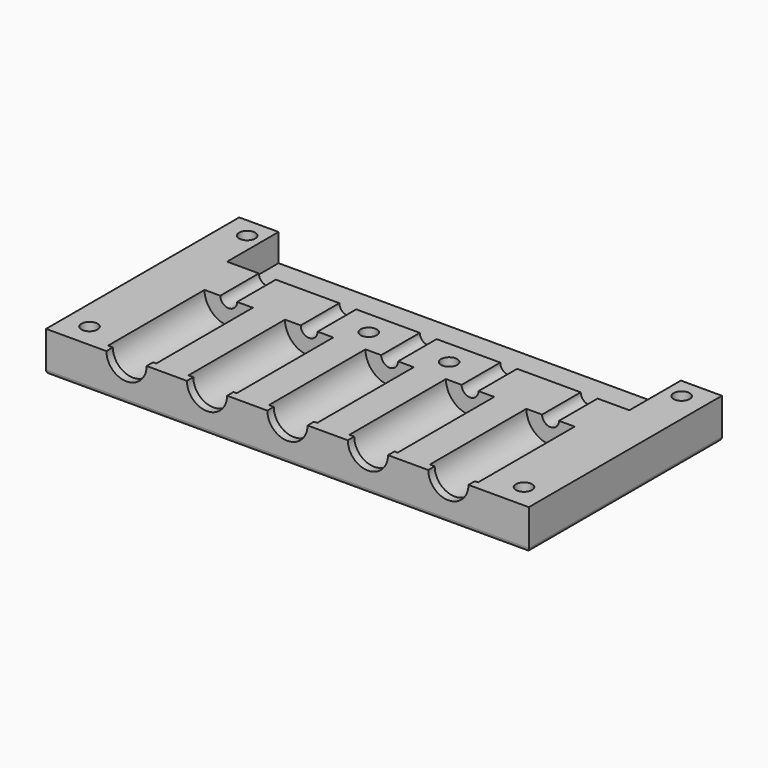
from build123d import *

# Parameters (mm, degrees)
F0_W      = 60
F0_H      = 25
F1_DEPTH  = 5
F2_R      = 2.5
F3_DEPTH  = 10
F5_R      = 3
F6_DEPTH  = 15
F7_R      = 1.05
F8_DEPTH  = 29
F9_W      = 50
F9_H      = 3.4154356362
F10_DEPTH = 3
F11_DEPTH = 5
F12_R     = 0.5
F14_R     = 1
F13_R     = 1
F15_DEPTH = 5.001
F16_R     = 1
F17_DEPTH = 5
F19_DEPTH = 1.5


with BuildPart() as f1:
    # F0 (on Top) → F1 (new body)
    with BuildSketch(Plane.XY):
        with Locations((-2.9453901201, -7.2920476746)):
            Rectangle(F0_W, F0_H)
    extrude(amount=F1_DEPTH)

    # F2 (on face) → F3 (cut)
    with BuildSketch(Plane.XZ.offset(19.7920476746)):
        with Locations((-22.9453901201, 5)):
            Circle(F2_R)
        with Locations((-12.9453901201, 5)):
            Circle(F2_R)
        with Locations((-2.9453901201, 5)):
            Circle(F2_R)
        with Locations((7.0546098799, 5)):
            Circle(F2_R)
        with Locations((17.0546098799, 5)):
            Circle(F2_R)
    extrude(amount=-F3_DEPTH, mode=Mode.SUBTRACT)

    # F5 (on offset) → F6 (cut)
    with BuildSketch(Plane.XZ.offset(18.7920476746)):
        with Locations((-23.0476632714, 5.0127296709)):
            Circle(F5_R)
        with Locations((-13.0476632714, 5.0127296709)):
            Circle(F5_R)
        with Locations((-3.0476632714, 5.0127296709)):
            Circle(F5_R)
        with Locations((6.9523367286, 5.0127296709)):
            Circle(F5_R)
        with Locations((16.9523367286, 5.0127296709)):
            Circle(F5_R)
    extrude(amount=-F6_DEPTH, mode=Mode.SUBTRACT)

    # F7 (on face) → F8 (cut)
    with BuildSketch(Plane.XZ.offset(3.7920476746)):
        with Locations((-23.0476632714, 5.0127296709)):
            Circle(F7_R)
        with Locations((-13.0476632714, 5.0127296709)):
            Circle(F7_R)
        with Locations((-3.0476632714, 5.0127296709)):
            Circle(F7_R)
        with Locations((6.9523367286, 5.0127296709)):
            Circle(F7_R)
        with Locations((16.9523367286, 5.0127296709)):
            Circle(F7_R)
    extrude(amount=-F8_DEPTH, mode=Mode.SUBTRACT)

    # F9 (on face) → F10 (cut)
    with BuildSketch(Plane(origin=(0, 5.2079523254, 0), x_dir=(-1, 0, 0), z_dir=(0, 1, 0))):
        with Locations((3.0476632714, 3.2922821819)):
            Rectangle(F9_W, F9_H)
    extrude(amount=-F10_DEPTH, mode=Mode.SUBTRACT)

    # F11 (add): a face of the model
    f11_faces = [f1.faces().sort_by_distance(p)[0] for p in [
        (-2.8102387692, 5.2079523254, 1.4530193808),
    ]]
    extrude(f11_faces, amount=F11_DEPTH)

    # F12
    f12_edges = [f1.edges().sort_by_distance(p)[0] for p in [
        (27.05461, -4.792048, 0),
        (-2.94539, -19.792048, 0),
        (-32.94539, -4.792048, 0),
    ]]
    fillet(f12_edges, radius=F12_R)

    # F14 (on face) + F13 (on face) → F15 (cut, through all)
    with BuildSketch(Plane(origin=(0, 0, 0), x_dir=(1, 0, 0), z_dir=(0, 0, -1))):
        with Locations((-29.9453901201, -7.7079523254)):
            Circle(F14_R)
        with Locations((24.0546098799, -7.7079523254)):
            Circle(F14_R)
    with BuildSketch(Plane(origin=(0, 0, 0), x_dir=(1, 0, 0), z_dir=(0, 0, -1))):
        with Locations((-29.9453901201, 16.7920476746)):
            Circle(F13_R)
        with Locations((24.0546098799, 16.7920476746)):
            Circle(F13_R)
    extrude(amount=-F15_DEPTH, mode=Mode.SUBTRACT)

    # F16 (on face) → F17 (cut)
    with BuildSketch(Plane.XY.offset(5)):
        with Locations((1.9524138955, -0.7920476746)):
            Circle(F16_R)
        with Locations((-8.0475861045, -0.7920476746)):
            Circle(F16_R)
    extrude(amount=-F17_DEPTH, mode=Mode.SUBTRACT)

    # F18 (on face) → F19 (cut)
    with BuildSketch(Plane(origin=(0, 0, 0), x_dir=(1, 0, 0), z_dir=(0, 0, -1))):
        Polygon((25.2093104182, -5.7079523254), (22.8999093415, -5.7079523254), (21.7452088031, -7.7079523254), (22.8999093415, -9.7079523254), (25.2093104182, -9.7079523254), (26.3640109566, -7.7079523254), align=None)
        Polygon((25.2093104182, 18.7920476746), (22.8999093415, 18.7920476746), (21.7452088031, 16.7920476746), (22.8999093415, 14.7920476746), (25.2093104182, 14.7920476746), (26.3640109566, 16.7920476746), align=None)
        Polygon((-28.7906895818, 18.7920476746), (-31.1000906585, 18.7920476746), (-32.2547911969, 16.7920476746), (-31.1000906585, 14.7920476746), (-28.7906895818, 14.7920476746), (-27.6359890434, 16.7920476746), align=None)
        Polygon((-31.1000906585, -9.7079523254), (-28.7906895818, -9.7079523254), (-27.6359890434, -7.7079523254), (-28.7906895818, -5.7079523254), (-31.1000906585, -5.7079523254), (-32.2547911969, -7.7079523254), align=None)
        Polygon((0.7977133571, -1.2079523254), (3.1071144338, -1.2079523254), (4.2618149722, 0.7920476746), (3.1071144338, 2.7920476746), (0.7977133571, 2.7920476746), (-0.3569871813, 0.7920476746), align=None)
        Polygon((-9.2022866429, -1.2079523254), (-6.8928855662, -1.2079523254), (-5.7381850278, 0.7920476746), (-6.8928855662, 2.7920476746), (-9.2022866429, 2.7920476746), (-10.3569871813, 0.7920476746), align=None)
    extrude(amount=-F19_DEPTH, mode=Mode.SUBTRACT)


solid = f1.part
